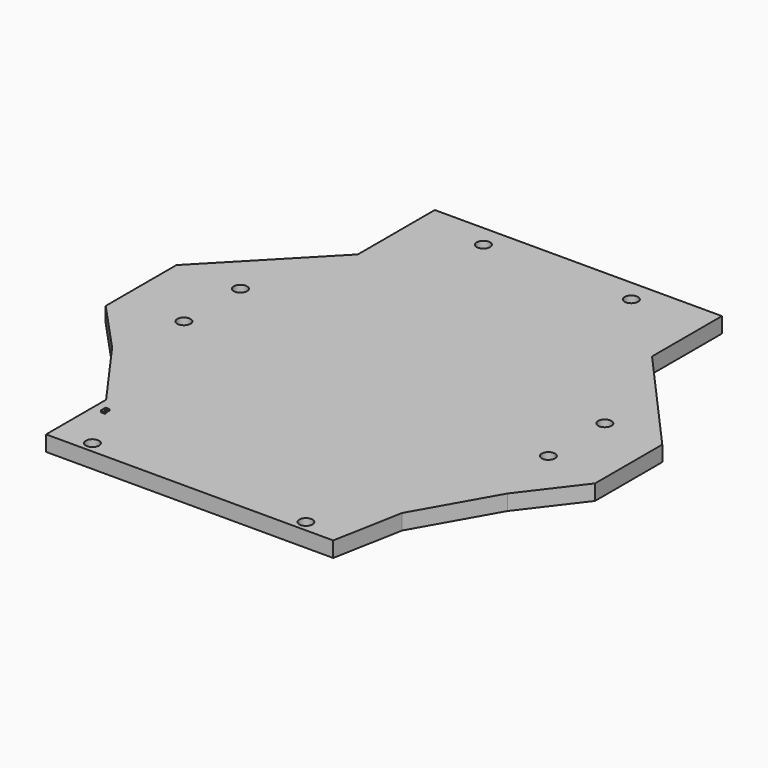
from build123d import *

# Parameters (mm, degrees)
F2_DEPTH    = 3.5
F3_R        = 1.5
F4_DEPTH    = 25
F5_W        = 15
F5_H        = 6
F6_DEPTH    = 28
F7_T1_DEPTH = 40
F8_W        = 0.6
F8_H        = 0.6
F9_DEPTH    = 0.39


# Not quite as in the source:
# - a fillet or chamfer that OpenCascade refuses, or shapes differently, is made with other operations: its cross-section is extruded or revolved along the edge and cut away or added


with BuildPart() as f2:
    # F0 (on Top) → F2 (new body)
    with BuildSketch(Plane.XY):
        Polygon((32.5, 70.6530249731), (-32.5, 70.6530249731), (-32.5, 59.4207410195), (-32.5, 48.8827627578), (-55, 25.6526721455), (-55, 5.6526721455), (-44.1446197954, -6.101506712), (-32.5, -22.3619750269), (-32.5, -39.3469750269), (32.5, -39.3469750269), (35.4572725267, -23.5087187488), (45.3055703038, -6.101506712), (55, 6.6271237275), (55, 25.6530249731), (32.5, 50.8760847151), align=None)
    extrude(amount=F2_DEPTH)

    # F3 (on face) → F4 (cut)
    with BuildSketch(Plane.XY.offset(3.5)):
        with Locations((-17.5, 65.6530249731)):
            Circle(F3_R)
        with Locations((16, 65.6530249731)):
            Circle(F3_R)
        with Locations((-40.5, 25.6526721455)):
            Circle(F3_R)
        with Locations((-40.5, 9.6526721455)):
            Circle(F3_R)
        with Locations((42, 25.6526721455)):
            Circle(F3_R)
        with Locations((42, 9.6526721455)):
            Circle(F3_R)
        with Locations((24.3198931655, -36.8469750269)):
            Circle(F3_R)
        with Locations((-24, -36.8469750269)):
            Circle(F3_R)
    extrude(amount=-F4_DEPTH, mode=Mode.SUBTRACT)

    # F5 (on face) → F6 (join)
    with BuildSketch(Plane.XY):
        with Locations((-0.6, 64.9171224535)):
            Rectangle(F5_W, F5_H)
    extrude(amount=-F6_DEPTH)

    # F7: fillet of radius 5 on 2 edges, made by hand

    # F7_s2 → F7_t1 (cut)
    with BuildSketch(Plane.YZ.offset(-20.6)):
        with BuildLine():
            ThreePointArc((61.9171224535, -23), (63.3815885475, -26.5355339059), (66.9171224535, -28))
            Line((66.9171224535, -28), (61.9171224535, -28))
            Line((61.9171224535, -28), (61.9171224535, -23))
        make_face()
        with BuildLine():
            ThreePointArc((67.9171224535, -23), (66.4526563594, -26.5355339059), (62.9171224535, -28))
            Line((62.9171224535, -28), (67.9171224535, -28))
            Line((67.9171224535, -28), (67.9171224535, -23))
        make_face()
    extrude(amount=F7_T1_DEPTH, mode=Mode.SUBTRACT)

    # F8 (on face) → F9 (join)
    with BuildSketch(Plane.XY.offset(3.5)):
        Polygon((-30.2116373062, -25.3581409693), (-30.2116373062, -25.5081409693), (-30.0116373062, -25.5081409693), (-29.9116373062, -25.5081409693), (-29.3116373062, -25.5081409693), (-29.3116373062, -25.3581409693), align=None)
        Polygon((-30.0116373062, -25.5081409693), (-30.2116373062, -25.5081409693), (-30.2116373062, -26.7081409693), (-29.9116373062, -26.7081409693), (-29.9116373062, -26.1081409693), (-29.9116373062, -25.5081409693), align=None)
        with Locations((-29.6116373062, -26.4081409693)):
            Rectangle(F8_W, F8_H)
    extrude(amount=F9_DEPTH)


solid = f2.part
